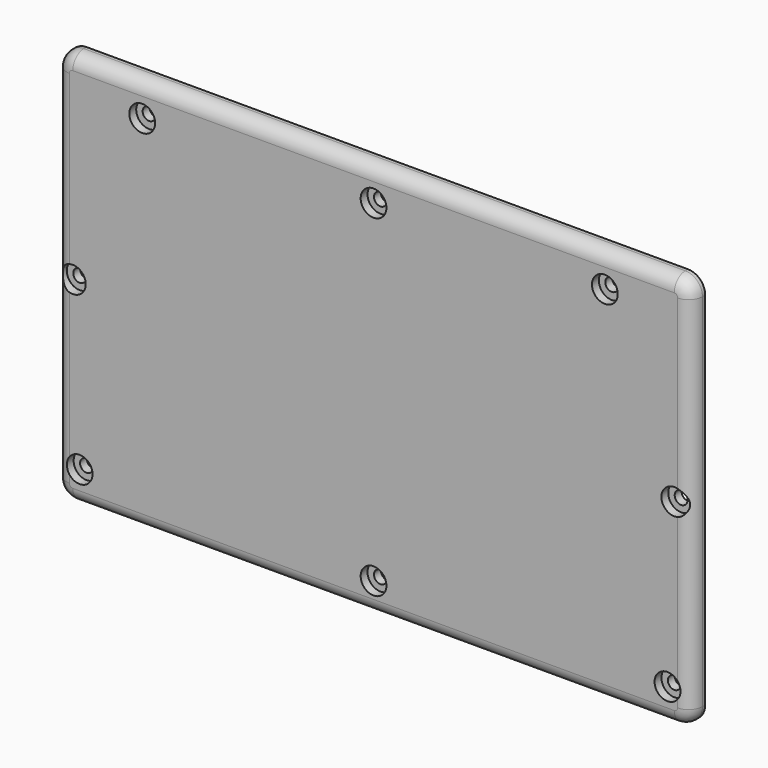
from build123d import *

# Parameters (mm, degrees)
F0_R         = 2.38125
F1_DEPTH     = 6.35
F2_R         = 4.7625
F3_DEPTH     = 3.175
F4_T1_DEPTH  = 133.35
F4_T3_DEPTH  = 222.25
F4_T6_ANGLE  = 90
F4_T8_ANGLE  = 90
F4_T10_ANGLE = 90
F4_T12_ANGLE = 90
F6_DEPTH     = 0.79375
F8_R         = 4.7625
F9_DEPTH     = 3.175


# Not quite as in the source:
# - a fillet or chamfer that OpenCascade refuses, or shapes differently, is made with other operations: its cross-section is extruded or revolved along the edge and cut away or added


with BuildPart() as f1:
    # F0 (on Front) → F1 (new body)
    with BuildSketch(Plane.XZ):
        with BuildLine():
            Line((123.8407226482, 73.3042017429), (-98.4092773518, 73.3042017429))
            ThreePointArc((-98.4092773518, 73.3042017429), (-102.8994054124, 71.4443298034), (-104.7592773518, 66.9542017429))
            Line((-104.7592773518, 66.9542017429), (-104.7592773518, -66.3957982571))
            ThreePointArc((-104.7592773518, -66.3957982571), (-102.8994054124, -70.8859263176), (-98.4092773518, -72.7457982571))
            Line((-98.4092773518, -72.7457982571), (123.8407226482, -72.7457982571))
            ThreePointArc((123.8407226482, -72.7457982571), (128.3308507087, -70.8859263176), (130.1907226482, -66.3957982571))
            Line((130.1907226482, -66.3957982571), (130.1907226482, 66.9542017429))
            ThreePointArc((130.1907226482, 66.9542017429), (128.3308507087, 71.4443298034), (123.8407226482, 73.3042017429))
        make_face()
        with Locations((-95.8918413821, -60.7033622874)):
            Circle(F0_R, mode=Mode.SUBTRACT)
        with Locations((12.7157226482, -61.6332982571)):
            Circle(F0_R, mode=Mode.SUBTRACT)
        with Locations((-98.4092773518, 0.2792017429)):
            Circle(F0_R, mode=Mode.SUBTRACT)
        with Locations((121.3232866785, -60.7033622874)):
            Circle(F0_R, mode=Mode.SUBTRACT)
        with Locations((123.8407226482, 0.2792017429)):
            Circle(F0_R, mode=Mode.SUBTRACT)
        with Locations((-72.7617797518, 61.2646017429)):
            Circle(F0_R, mode=Mode.SUBTRACT)
        with Locations((12.7157226482, 61.2646017429)):
            Circle(F0_R, mode=Mode.SUBTRACT)
        with Locations((98.1932250482, 61.2646017429)):
            Circle(F0_R, mode=Mode.SUBTRACT)
    extrude(amount=F1_DEPTH)

    # F2 (on face) → F3 (cut)
    with BuildSketch(Plane.XZ.offset(6.35)):
        with Locations((12.7157226482, 61.2646017429)):
            Circle(F2_R)
        with Locations((123.8407226482, 0.2792017429)):
            Circle(F2_R)
        with Locations((121.3232866785, -60.7033622874)):
            Circle(F2_R)
        with Locations((12.7157226482, -61.6332982571)):
            Circle(F2_R)
        with Locations((-95.8918413821, -60.7033622874)):
            Circle(F2_R)
        with Locations((-98.4092773518, 0.2792017429)):
            Circle(F2_R)
    extrude(amount=-F3_DEPTH, mode=Mode.SUBTRACT)

    # F4: fillet of radius 5.08 on 8 edges, made by hand

    # F4_s2 → F4_t1 (cut)
    with BuildSketch(Plane.XY.offset(-66.3957982571)):
        with BuildLine():
            ThreePointArc((-99.6792773518, -6.35), (-103.2713798002, -4.8621024484), (-104.7592773518, -1.27))
            Line((-104.7592773518, -1.27), (-104.7592773518, -6.35))
            Line((-104.7592773518, -6.35), (-99.6792773518, -6.35))
        make_face()
        with BuildLine():
            ThreePointArc((130.1907226482, -1.27), (128.7028250966, -4.8621024484), (125.1107226482, -6.35))
            Line((125.1107226482, -6.35), (130.1907226482, -6.35))
            Line((130.1907226482, -6.35), (130.1907226482, -1.27))
        make_face()
    extrude(amount=F4_T1_DEPTH, mode=Mode.SUBTRACT)

    # F4_s4 → F4_t3 (cut)
    with BuildSketch(Plane.YZ.offset(-98.4092773518)):
        with BuildLine():
            ThreePointArc((-1.27, 73.3042017429), (-4.8621024484, 71.8163041913), (-6.35, 68.2242017429))
            Line((-6.35, 68.2242017429), (-6.35, 73.3042017429))
            Line((-6.35, 73.3042017429), (-1.27, 73.3042017429))
        make_face()
        with BuildLine():
            ThreePointArc((-6.35, -67.6657982571), (-4.8621024484, -71.2579007055), (-1.27, -72.7457982571))
            Line((-1.27, -72.7457982571), (-6.35, -72.7457982571))
            Line((-6.35, -72.7457982571), (-6.35, -67.6657982571))
        make_face()
    extrude(amount=F4_T3_DEPTH, mode=Mode.SUBTRACT)

    # F4_s5 → F4_t6 (revolve, cut)
    with BuildSketch(Plane.YZ.offset(-98.4092773518)):
        with BuildLine():
            ThreePointArc((-6.35, 68.2242017429), (-4.8621024484, 71.8163041913), (-1.27, 73.3042017429))
            Line((-1.27, 73.3042017429), (-6.35, 73.3042017429))
            Line((-6.35, 73.3042017429), (-6.35, 68.2242017429))
        make_face()
    revolve(axis=Axis((-98.4092773518, -6.35, 66.9542017429), (0, -1, 0)), revolution_arc=F4_T6_ANGLE, mode=Mode.SUBTRACT)

    # F4_s7 → F4_t8 (revolve, cut)
    with BuildSketch(Plane.XY.offset(66.9542017429)):
        with BuildLine():
            ThreePointArc((130.1907226482, -1.27), (128.7028250966, -4.8621024484), (125.1107226482, -6.35))
            Line((125.1107226482, -6.35), (130.1907226482, -6.35))
            Line((130.1907226482, -6.35), (130.1907226482, -1.27))
        make_face()
    revolve(axis=Axis((123.8407226482, -6.35, 66.9542017429), (0, -1, 0)), revolution_arc=F4_T8_ANGLE, mode=Mode.SUBTRACT)

    # F4_s9 → F4_t10 (revolve, cut)
    with BuildSketch(Plane.YZ.offset(123.8407226482)):
        with BuildLine():
            ThreePointArc((-6.35, -67.6657982571), (-4.8621024484, -71.2579007055), (-1.27, -72.7457982571))
            Line((-1.27, -72.7457982571), (-6.35, -72.7457982571))
            Line((-6.35, -72.7457982571), (-6.35, -67.6657982571))
        make_face()
    revolve(axis=Axis((123.8407226482, -6.35, -66.3957982571), (0, -1, 0)), revolution_arc=F4_T10_ANGLE, mode=Mode.SUBTRACT)

    # F4_s11 → F4_t12 (revolve, cut)
    with BuildSketch(Plane.XY.offset(-66.3957982571)):
        with BuildLine():
            ThreePointArc((-99.6792773518, -6.35), (-103.2713798002, -4.8621024484), (-104.7592773518, -1.27))
            Line((-104.7592773518, -1.27), (-104.7592773518, -6.35))
            Line((-104.7592773518, -6.35), (-99.6792773518, -6.35))
        make_face()
    revolve(axis=Axis((-98.4092773518, -6.35, -66.3957982571), (0, -1, 0)), revolution_arc=F4_T12_ANGLE, mode=Mode.SUBTRACT)

    # F5 (on face) → F6 (join)
    with BuildSketch(Plane.XZ):
        with BuildLine():
            Line((-92.0592773518, 47.9042017429), (-92.0592773518, -47.3457982571))
            ThreePointArc((-92.0592773518, -47.3457982571), (-90.1994054124, -51.8359263176), (-85.7092773518, -53.6957982571))
            Line((-85.7092773518, -53.6957982571), (111.1407226482, -53.6957982571))
            ThreePointArc((111.1407226482, -53.6957982571), (115.6308507087, -51.8359263176), (117.4907226482, -47.3457982571))
            Line((117.4907226482, -47.3457982571), (117.4907226482, 47.9042017429))
            ThreePointArc((117.4907226482, 47.9042017429), (115.6308507087, 52.3943298034), (111.1407226482, 54.2542017429))
            Line((111.1407226482, 54.2542017429), (-85.7092773518, 54.2542017429))
            ThreePointArc((-85.7092773518, 54.2542017429), (-90.1994054124, 52.3943298034), (-92.0592773518, 47.9042017429))
        make_face()
        with BuildLine():
            ThreePointArc((-88.8842773518, 47.9042017429), (-87.9543413821, 50.1492657732), (-85.7092773518, 51.0792017429))
            Line((-85.7092773518, 51.0792017429), (111.1407226482, 51.0792017429))
            ThreePointArc((111.1407226482, 51.0792017429), (113.3857866785, 50.1492657732), (114.3157226482, 47.9042017429))
            Line((114.3157226482, 47.9042017429), (114.3157226482, -47.3457982571))
            ThreePointArc((114.3157226482, -47.3457982571), (113.3857866785, -49.5908622874), (111.1407226482, -50.5207982571))
            Line((111.1407226482, -50.5207982571), (-85.7092773518, -50.5207982571))
            ThreePointArc((-85.7092773518, -50.5207982571), (-87.9543413821, -49.5908622874), (-88.8842773518, -47.3457982571))
            Line((-88.8842773518, -47.3457982571), (-88.8842773518, 47.9042017429))
        make_face(mode=Mode.SUBTRACT)
    extrude(amount=-F6_DEPTH)

    # F8 (on face) → F9 (cut)
    with BuildSketch(Plane.XZ.offset(6.35)):
        with Locations((-72.7617797518, 61.0206037701)):
            Circle(F8_R)
        with Locations((98.1932250482, 61.0206037701)):
            Circle(F8_R)
    extrude(amount=-F9_DEPTH, mode=Mode.SUBTRACT)


solid = f1.part
